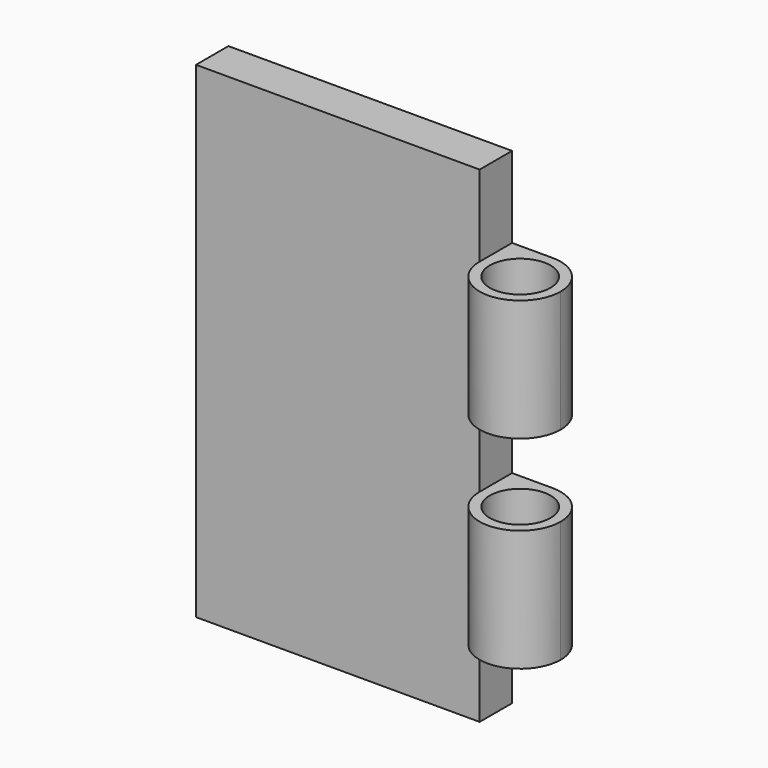
from build123d import *

# Parameters (mm, degrees)
F0_W     = 101.6
F0_H     = 152.4
F1_DEPTH = 12.7
F3_DEPTH = 152.4
F4_R     = 9.525
F5_DEPTH = 152.4
F7_W     = 50.8
F7_H     = 25.4
F8_DEPTH = 50.8


# Not quite as in the source:
# - a feature names something its author has since deleted; it is built from what else it names


with BuildPart() as f1:
    # F0 (on Front) → F1 (new body)
    with BuildSketch(Plane.XZ):
        with Locations((11.3006858155, 1.2977712616)):
            Rectangle(F0_W, F0_H)
    extrude(amount=F1_DEPTH)

    # F2 (on face) → F3 (join)
    with BuildSketch(Plane.XY.offset(77.4977712616)):
        with BuildLine():
            ThreePointArc((49.4006858155, -12.7), (62.1006858155, -25.4), (74.8006858155, -12.7))
            ThreePointArc((74.8006858155, -12.7), (71.0809419366, -3.7197438789), (62.1006858155, 0))
            Line((62.1006858155, 0), (62.1006858155, -12.7))
            Line((62.1006858155, -12.7), (49.4006858155, -12.7))
        make_face()
    extrude(amount=-F3_DEPTH)

    # F4 (on face) → F5 (cut, through all)
    with BuildSketch(Plane.XY.offset(77.4977712616)):
        with Locations((62.1006858155, -12.7)):
            Circle(F4_R)
    extrude(amount=-F5_DEPTH, mode=Mode.SUBTRACT)

    # F7 (on offset) → F8 (cut)
    with BuildSketch(Plane.XZ.offset(25.4)):
        with Locations((74.8006858155, 64.7977712616)):
            Rectangle(F7_W, F7_H)
        with Locations((74.8006858155, -62.2022287384)):
            Rectangle(F7_W, F7_H)
        with Locations((74.8006858155, 1.2977712616)):
            Rectangle(F7_W, F7_H)
    extrude(amount=-F8_DEPTH, mode=Mode.SUBTRACT)


solid = f1.part
